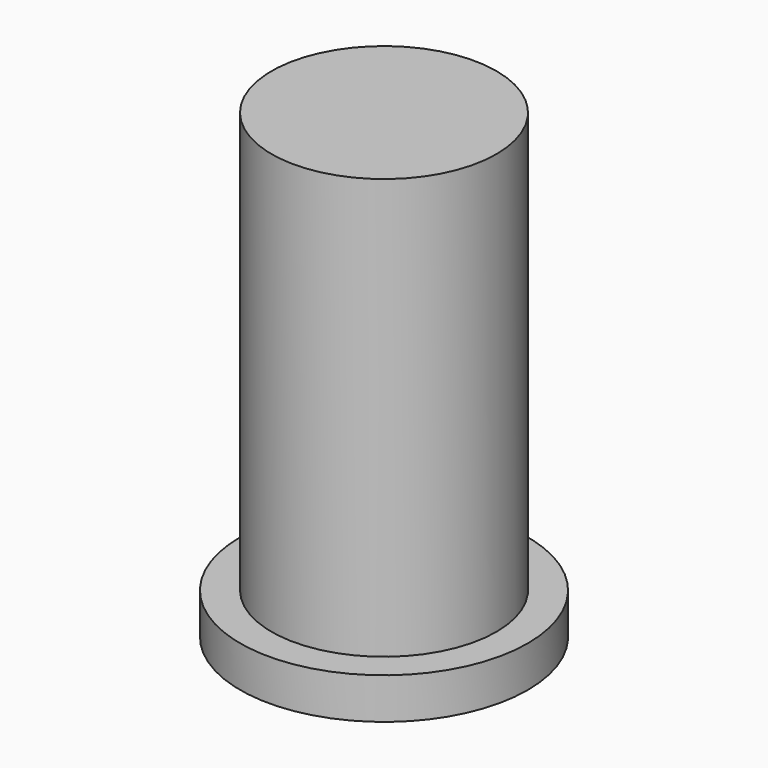
from build123d import *

# Parameters (mm, degrees)
F0_R     = 5.75
F1_DEPTH = 21.5
F2_R     = 7.35
F2_R_2   = 5.75
F3_DEPTH = 2.1


with BuildPart() as f1:
    # F0 (on Top) → F1 (new body)
    with BuildSketch(Plane.XY):
        Circle(F0_R)
    extrude(amount=F1_DEPTH)

    # F2 (on face) → F3 (join)
    with BuildSketch(Plane(origin=(0, 0, 0), x_dir=(1, 0, 0), z_dir=(0, 0, -1))):
        Circle(F2_R)
        Circle(F2_R_2, mode=Mode.SUBTRACT)
        Circle(F2_R_2)
    extrude(amount=F3_DEPTH)


solid = f1.part
